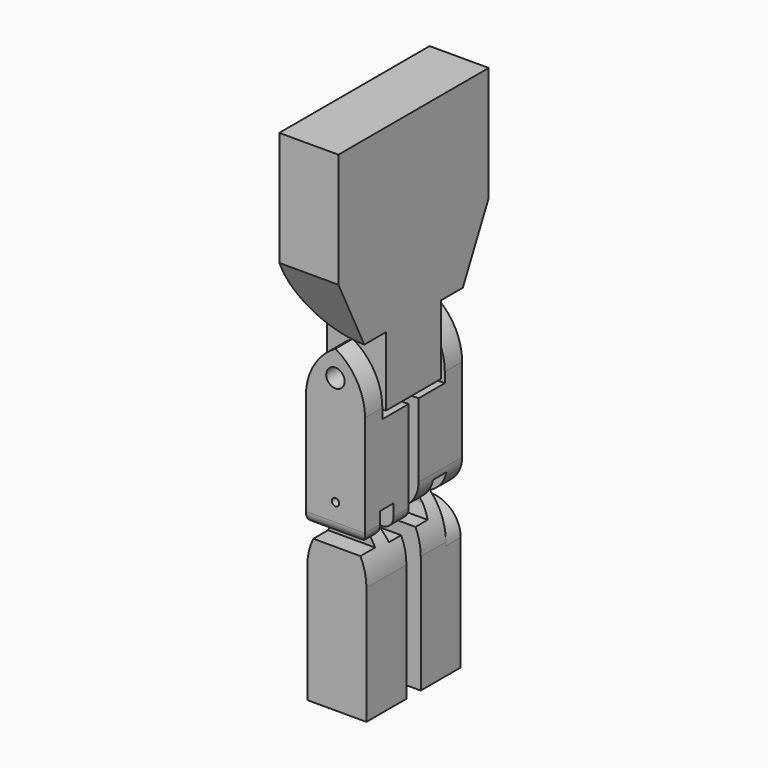
from build123d import *

# Parameters (mm, degrees)
F6_DEPTH       = 12.7
F7_DEPTH       = 12.7
F8_DEPTH       = 12.7
F9_F1_R        = 12.7
F9_F2_R        = 12.6999
F9_2_T1_DEPTH  = 71.6003941596
F9_2_T3_DEPTH  = 71.6003969535
F10_R          = 5.08
F11_T1_DEPTH   = 132.8857165277
F11_2_T1_DEPTH = 132.8857165277
F12_T1_DEPTH   = 136.3004535884
F12_2_T1_DEPTH = 136.3004535884
F12_3_F1_R     = 25.3999
F12_3_F2_R     = 25.3999
F13_R          = 3.1967586716
F14_DEPTH      = 40.3502301702
F15_R          = 3.9621319953
F16_DEPTH      = 66.4104053209
F19_R          = 1.5875
F20_DEPTH      = 66.4104053209


# Not quite as in the source:
# - a fillet or chamfer that OpenCascade refuses, or shapes differently, is made with other operations: its cross-section is extruded or revolved along the edge and cut away or added
# - a fillet or chamfer is up to 0.001 mm smaller than in the source, because OpenCascade refuses the exact size
# - a feature of the source that left no trace in its solid (it failed there, or was rolled back) is left out
# - the program builds the solid bodies; features that only make, move or delete a surface that nothing else refers to are left out


with BuildPart() as f6:
    # F5 (on Right) → F6 (new body, symmetric)
    with BuildSketch(Plane.YZ):
        Polygon((17.381310463, -124.0725144744), (17.381310463, -114.1014173627), (11.4955939353, -114.1014173627), (11.4955939353, -123.9340305328), (10.4060629383, -129.0555149317), (3.8553033955, -129.0555149317), (3.8553033955, -190.1959329844), (8.2224793732, -190.1959329844), (20.4505622387, -190.1959329844), (25.3053139895, -190.1959329844), (25.3053139895, -128.343090415), (17.381310463, -128.343090415), align=None)
    extrude(amount=F6_DEPTH, both=True)

    # F9: fillet of radius 12.7 on 2 edges, made by hand

    # F9_f1
    f9_f1_edges = [f6.edges().sort_by_distance(p)[0] for p in [
        (-12.7, 21.3433122262, -128.343090415),
    ]]
    fillet(f9_f1_edges, radius=F9_F1_R)

    # F9_f2 (radius 12.7 in the source; OpenCascade refuses exactly that, so slightly less here)
    f9_f2_edges = [f6.edges().sort_by_distance(p)[0] for p in [
        (12.7, 21.3433122262, -128.343090415),
    ]]
    fillet(f9_f2_edges, radius=F9_F2_R)

    # F11: fillet of radius 25.4 on 2 edges, made by hand

    # F11_s2 → F11_t1 (cut)
    with BuildSketch(Plane.XZ.offset(-80.881310463)):
        with BuildLine():
            ThreePointArc((12.7, -139.5014173627), (5.2605122421, -121.5409051206), (-12.7, -114.1014173627))
            Line((-12.7, -114.1014173627), (12.7, -114.1014173627))
            Line((12.7, -114.1014173627), (12.7, -139.5014173627))
        make_face()
        with BuildLine():
            ThreePointArc((-12.7, -139.5014173627), (-5.2605122421, -121.5409051206), (12.7, -114.1014173627))
            Line((12.7, -114.1014173627), (-12.7, -114.1014173627))
            Line((-12.7, -114.1014173627), (-12.7, -139.5014173627))
        make_face()
    extrude(amount=F11_T1_DEPTH, mode=Mode.SUBTRACT)


with BuildPart() as f6b:
    # F5 (on Right) → F6, piece 2 (new body, symmetric)
    with BuildSketch(Plane.YZ):
        Polygon((-17.381310463, -128.343090415), (-25.3053139895, -128.343090415), (-25.3053139895, -190.1959329844), (-20.4505622387, -190.1959329844), (-8.2224793732, -190.1959329844), (-3.8553033955, -190.1959329844), (-3.8553033955, -129.0555149317), (-10.4060629383, -129.0555149317), (-11.4955939353, -123.9340305328), (-11.4955939353, -114.1014173627), (-17.381310463, -114.1014173627), (-17.381310463, -124.0725144744), align=None)
    extrude(amount=F6_DEPTH, both=True)

    # F11#2: fillet of radius 25.4 on 2 edges, made by hand

    # F11_2_s2 → F11_2_t1 (cut)
    with BuildSketch(Plane.XZ.offset(-52.0044060647)):
        with BuildLine():
            ThreePointArc((-12.7, -114.1014173627), (5.2605122421, -121.5409051206), (12.7, -139.5014173627))
            Line((12.7, -139.5014173627), (12.7, -114.1014173627))
            Line((12.7, -114.1014173627), (-12.7, -114.1014173627))
        make_face()
        with BuildLine():
            ThreePointArc((12.7, -114.1014173627), (-5.2605122421, -121.5409051206), (-12.7, -139.5014173627))
            Line((-12.7, -139.5014173627), (-12.7, -114.1014173627))
            Line((-12.7, -114.1014173627), (12.7, -114.1014173627))
        make_face()
    extrude(amount=F11_2_T1_DEPTH, mode=Mode.SUBTRACT)


with BuildPart() as f7:
    # F4 (on Right) → F7 (new body, symmetric)
    with BuildSketch(Plane.YZ):
        Polygon((26.0601751506, -123.6367598176), (26.0601751506, -49.5331436396), (16.7597215623, -49.5331436396), (16.7597215623, -79.2345926166), (2.65903119, -79.2345926166), (2.65903119, -123.6367598176), (10.7594281435, -123.6367598176), (10.7594281435, -113.4362667799), (17.9597809911, -113.4362667799), (17.9597809911, -123.6367598176), align=None)
    extrude(amount=F7_DEPTH, both=True)

    # F9#2: fillet of radius 12.7 on 4 edges, made by hand

    # F9_2_s2 → F9_2_t1 (cut)
    with BuildSketch(Plane.XZ.offset(-57.8101751506)):
        with BuildLine():
            ThreePointArc((0, -123.6367598176), (8.9802561211, -119.9170159387), (12.7, -110.9367598176))
            Line((12.7, -110.9367598176), (12.7, -123.6367598176))
            Line((12.7, -123.6367598176), (0, -123.6367598176))
        make_face()
        with BuildLine():
            ThreePointArc((0, -123.6367598176), (-8.9802561211, -119.9170159387), (-12.7, -110.9367598176))
            Line((-12.7, -110.9367598176), (-12.7, -123.6367598176))
            Line((-12.7, -123.6367598176), (0, -123.6367598176))
        make_face()
    extrude(amount=F9_2_T1_DEPTH, mode=Mode.SUBTRACT)

    # F9_2_s4 → F9_2_t3 (cut)
    with BuildSketch(Plane.XZ.offset(-42.5094281435)):
        with BuildLine():
            ThreePointArc((0, -123.6367598176), (-8.9802561211, -119.9170159387), (-12.7, -110.9367598176))
            Line((-12.7, -110.9367598176), (-12.7, -123.6367598176))
            Line((-12.7, -123.6367598176), (0, -123.6367598176))
        make_face()
        with BuildLine():
            ThreePointArc((0, -123.6367598176), (8.9802561211, -119.9170159387), (12.7, -110.9367598176))
            Line((12.7, -110.9367598176), (12.7, -123.6367598176))
            Line((12.7, -123.6367598176), (0, -123.6367598176))
        make_face()
    extrude(amount=F9_2_T3_DEPTH, mode=Mode.SUBTRACT)

    # F12: fillet of radius 25.4 on 2 edges, made by hand

    # F12_s2 → F12_t1 (cut)
    with BuildSketch(Plane.XZ.offset(-89.5601751506)):
        with BuildLine():
            ThreePointArc((12.7, -49.5331436396), (-5.2605122421, -56.9726313974), (-12.7, -74.9331436396))
            Line((-12.7, -74.9331436396), (-12.7, -49.5331436396))
            Line((-12.7, -49.5331436396), (12.7, -49.5331436396))
        make_face()
        with BuildLine():
            ThreePointArc((12.7, -74.9331436396), (5.2605122421, -56.9726313974), (-12.7, -49.5331436396))
            Line((-12.7, -49.5331436396), (12.7, -49.5331436396))
            Line((12.7, -49.5331436396), (12.7, -74.9331436396))
        make_face()
    extrude(amount=F12_T1_DEPTH, mode=Mode.SUBTRACT)


with BuildPart() as f7b:
    # F4 (on Right) → F7, piece 2 (new body, symmetric)
    with BuildSketch(Plane.YZ):
        Polygon((-16.7597215623, -49.5331436396), (-26.0601751506, -49.5331436396), (-26.0601751506, -123.6367598176), (-17.9597809911, -123.6367598176), (-17.9597809911, -113.4362667799), (-10.7594281435, -113.4362667799), (-10.7594281435, -123.6367598176), (-2.65903119, -123.6367598176), (-2.65903119, -79.2345926166), (-16.7597215623, -79.2345926166), align=None)
    extrude(amount=F7_DEPTH, both=True)

    # F10
    f10_edges = [f7b.edges().sort_by_distance(p)[0] for p in [
        (12.7, -22.009978, -123.63676),
        (0, -26.060175, -123.63676),
        (-12.7, -6.70923, -123.63676),
        (12.7, -6.70923, -123.63676),
    ]]
    fillet(f10_edges, radius=F10_R)

    # F12#2: fillet of radius 25.4 on 2 edges, made by hand

    # F12_2_s2 → F12_2_t1 (cut)
    with BuildSketch(Plane.XZ.offset(-46.7402784377)):
        with BuildLine():
            ThreePointArc((-12.7, -74.9331436396), (-5.2605122421, -56.9726313974), (12.7, -49.5331436396))
            Line((12.7, -49.5331436396), (-12.7, -49.5331436396))
            Line((-12.7, -49.5331436396), (-12.7, -74.9331436396))
        make_face()
        with BuildLine():
            ThreePointArc((12.7, -74.9331436396), (5.2605122421, -56.9726313974), (-12.7, -49.5331436396))
            Line((-12.7, -49.5331436396), (12.7, -49.5331436396))
            Line((12.7, -49.5331436396), (12.7, -74.9331436396))
        make_face()
    extrude(amount=F12_2_T1_DEPTH, mode=Mode.SUBTRACT)


with BuildPart() as f8:
    # F3 (on Right) → F8 (new body, symmetric)
    with BuildSketch(Plane.YZ):
        Polygon((40.3492301702, 30.3626544774), (-40.3492301702, 30.3626544774), (-40.3492301702, 0), (-40.3492301702, -18.7984760851), (-26.4357030392, -47.0893159509), (-14.841097407, -47.0893159509), (-14.841097407, -76.7751282773), (14.841097407, -76.7751282773), (14.841097407, -47.0893159509), (26.4357030392, -47.0893159509), (40.3492301702, -18.7984760851), (40.3492301702, 0), align=None)
    extrude(amount=F8_DEPTH, both=True)

    # F12#3: fillet of radius 25.4 on 2 edges, made by hand

    # F12_3_f1 (radius 25.4 in the source; OpenCascade refuses exactly that, so slightly less here)
    f12_3_f1_edges = [f8.edges().sort_by_distance(p)[0] for p in [
        (-12.7, 20.6384002231, -47.0893159509),
    ]]
    fillet(f12_3_f1_edges, radius=F12_3_F1_R)

    # F12_3_f2 (radius 25.4 in the source; OpenCascade refuses exactly that, so slightly less here)
    f12_3_f2_edges = [f8.edges().sort_by_distance(p)[0] for p in [
        (-12.7, -20.6384002231, -47.0893159509),
    ]]
    fillet(f12_3_f2_edges, radius=F12_3_F2_R)


with BuildPart() as f14_tool:
    # F13 (on Front) → F14 (new body, through all)
    with BuildSketch(Plane.XZ):
        with Locations((0, -63.4542033076)):
            Circle(F13_R)
    extrude(amount=-F14_DEPTH)


with BuildPart() as f7_1:
    add(f7.part)

    # F14: cut by f14_tool
    add(f14_tool.part, mode=Mode.SUBTRACT)


with BuildPart() as f8_1:
    add(f8.part)

    # F14: cut by f14_tool
    add(f14_tool.part, mode=Mode.SUBTRACT)


with BuildPart() as f16_tool:
    # F15 (on face) → F16 (new body, through all)
    with BuildSketch(Plane.XZ.offset(26.0601751506)):
        with Locations((0, -64.0083104372)):
            Circle(F15_R)
    extrude(amount=-F16_DEPTH)


with BuildPart() as f7_2:
    add(f7_1.part)

    # F16: cut by f16_tool
    add(f16_tool.part, mode=Mode.SUBTRACT)


with BuildPart() as f7b_1:
    add(f7b.part)

    # F16: cut by f16_tool
    add(f16_tool.part, mode=Mode.SUBTRACT)


with BuildPart() as f8_2:
    add(f8_1.part)

    # F16: cut by f16_tool
    add(f16_tool.part, mode=Mode.SUBTRACT)


with BuildPart() as f20_tool:
    # F19 (on face) → F20 (new body, through all)
    with BuildSketch(Plane.XZ.offset(26.0601751506)):
        with Locations((0, -110.9367598176)):
            Circle(F19_R)
    extrude(amount=-F20_DEPTH)


with BuildPart() as f7_3:
    add(f7_2.part)

    # F20: cut by f20_tool
    add(f20_tool.part, mode=Mode.SUBTRACT)


with BuildPart() as f7b_2:
    add(f7b_1.part)

    # F20: cut by f20_tool
    add(f20_tool.part, mode=Mode.SUBTRACT)


solid = Compound([f6.part, f6b.part, f8_2.part, f7_3.part, f7b_2.part])
